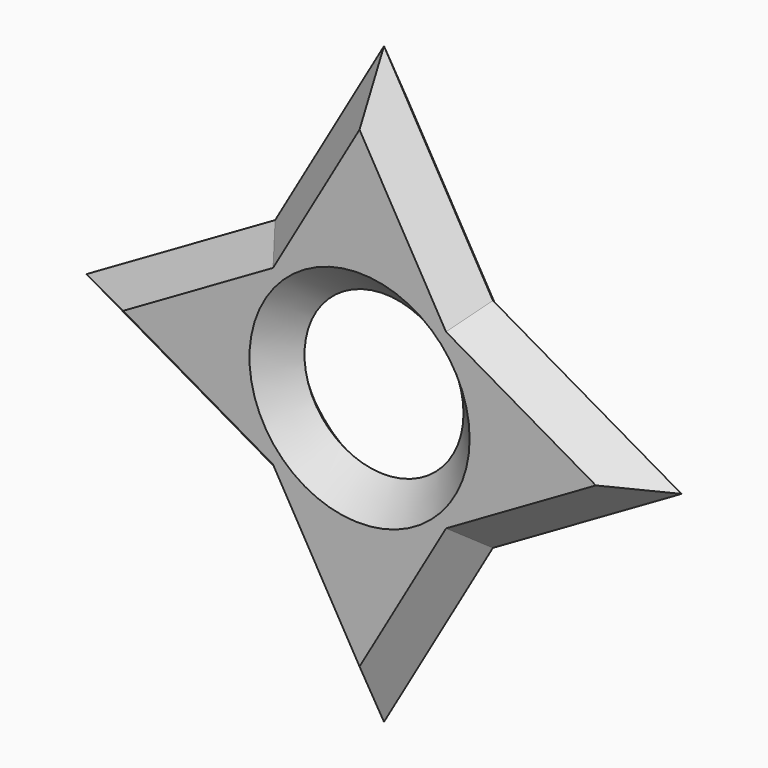
from build123d import *

# Parameters (mm, degrees)
F0_W         = 25.4
F0_H         = 25.4
F0_R         = 6.35
F1_DEPTH     = 6.35
F2_SIZE      = 5.08
F3_T4_DEPTH  = 51.5282991577
F3_T9_DEPTH  = 51.5282991577
F3_T14_DEPTH = 51.5282991577
F3_T19_DEPTH = 51.5282991577
F3_T24_DEPTH = 51.5282991577
F3_T29_DEPTH = 51.5282991577
F3_T34_DEPTH = 51.5282991577
F3_T39_DEPTH = 51.5282991577
F3_T47_DEPTH = 51.5282991577
F3_T51_DEPTH = 51.5282991577
F3_T58_DEPTH = 51.5282991577
F3_T62_DEPTH = 51.5282991577
F3_T69_DEPTH = 51.5282991577
F3_T73_DEPTH = 51.5282991577
F3_T80_DEPTH = 51.5282991577
F3_T84_DEPTH = 51.5282991577


# Not quite as in the source:
# - a fillet or chamfer that OpenCascade refuses, or shapes differently, is made with other operations: its cross-section is extruded or revolved along the edge and cut away or added


with BuildPart() as f1:
    # F0 (on Front) → F1 (new body)
    with BuildSketch(Plane.XZ):
        with Locations((12.7, 12.7)):
            Rectangle(F0_W, F0_H)
        with Locations((12.7, 12.7)):
            Circle(F0_R, mode=Mode.SUBTRACT)
        Polygon((12.7, 47.3970452561), (0, 25.4), (25.4, 25.4), align=None)
        Polygon((-21.9970452561, 12.7), (0, 0), (0, 25.4), align=None)
        Polygon((25.4, 25.4), (25.4, 0), (47.3970452561, 12.7), align=None)
        Polygon((25.4, 0), (0, 0), (12.7, -21.9970452561), align=None)
    extrude(amount=F1_DEPTH)

    # F2
    f2_edges = [f1.edges().sort_by_distance(p)[0] for p in [
        (36.398523, -6.35, 6.35),
        (36.398523, -6.35, 19.05),
        (19.05, -6.35, 36.398523),
        (6.35, -6.35, 36.398523),
        (-10.998523, -6.35, 19.05),
        (-10.998523, -6.35, 6.35),
        (6.35, -6.35, -10.998523),
        (19.05, -6.35, -10.998523),
        (6.35, -6.35, 12.7),
    ]]
    chamfer(f2_edges, length=F2_SIZE)

    # F3: chamfer of 5.08 on 9 edges, made by hand


with BuildPart() as f3_tool2:
    # F3_s3 → F3_t4 (new body)
    with BuildSketch(Plane(origin=(7.7361145859, 0, 4.4664478386), x_dir=(0, 1, 0), z_dir=(0.8660254038, 0, 0.5))):
        Polygon((-5.08, -12.7), (0, -7.62), (0, -12.7), align=None)
    extrude(amount=F3_T4_DEPTH)

    split(bisect_by=Plane(origin=(19.05, 0, -10.9985226281), x_dir=(0, 1, 0), z_dir=(0.8660254038, 0, -0.5)), keep=Keep.TOP)


with BuildPart() as f1_1:
    add(f1.part)

    # F3_t1: cut F3_tool2
    add(f3_tool2.part, mode=Mode.SUBTRACT)


with BuildPart() as f3_tool7:
    # F3_s8 → F3_t9 (new body)
    with BuildSketch(Plane(origin=(41.3624080422, 0, -23.8805974175), x_dir=(0, 1, 0), z_dir=(-0.8660254038, 0, 0.5))):
        Polygon((0, -29.6170452561), (-5.08, -34.6970452561), (0, -34.6970452561), align=None)
    extrude(amount=F3_T9_DEPTH)

    split(bisect_by=Plane(origin=(30.0485226281, 0, 17.3485226281), x_dir=(0, 1, 0), z_dir=(0.8660254038, 0, 0.5)), keep=Keep.TOP)


with BuildPart() as f1_2:
    add(f1_1.part)

    # F3_t6: cut F3_tool7
    add(f3_tool7.part, mode=Mode.SUBTRACT)


with BuildPart() as f3_tool12:
    # F3_s13 → F3_t14 (new body)
    with BuildSketch(Plane(origin=(1.8835521614, 0, -3.2624080422), x_dir=(0, 1, 0), z_dir=(-0.5, 0, 0.8660254038))):
        Polygon((0, -29.6170452561), (-5.08, -34.6970452561), (0, -34.6970452561), align=None)
    extrude(amount=F3_T14_DEPTH)

    split(bisect_by=Plane(origin=(17.3485226281, 0, 30.0485226281), x_dir=(0, 1, 0), z_dir=(0.5, 0, 0.8660254038)), keep=Keep.TOP)


with BuildPart() as f1_3:
    add(f1_2.part)

    # F3_t11: cut F3_tool12
    add(f3_tool12.part, mode=Mode.SUBTRACT)


with BuildPart() as f3_tool17:
    # F3_s18 → F3_t19 (new body)
    with BuildSketch(Plane(origin=(30.2305974175, 0, 52.3609306703), x_dir=(0, 1, 0), z_dir=(-0.5, 0, -0.8660254038))):
        Polygon((0, -7.62), (-5.08, -12.7), (0, -12.7), align=None)
    extrude(amount=F3_T19_DEPTH)

    split(bisect_by=Plane(origin=(-10.9985226281, 0, 19.05), x_dir=(0, 1, 0), z_dir=(-0.5, 0, 0.8660254038)), keep=Keep.TOP)


with BuildPart() as f1_4:
    add(f1_3.part)

    # F3_t16: cut F3_tool17
    add(f3_tool17.part, mode=Mode.SUBTRACT)


with BuildPart() as f3_tool22:
    # F3_s23 → F3_t24 (new body)
    with BuildSketch(Plane(origin=(22.3124080422, 0, 12.8820747894), x_dir=(0, 1, 0), z_dir=(-0.8660254038, 0, -0.5))):
        Polygon((0, -16.9170452561), (-5.08, -21.9970452561), (0, -21.9970452561), align=None)
    extrude(amount=F3_T24_DEPTH)

    split(bisect_by=Plane(origin=(-10.9985226281, 0, 6.35), x_dir=(0, 1, 0), z_dir=(-0.8660254038, 0, 0.5)), keep=Keep.TOP)


with BuildPart() as f1_5:
    add(f1_4.part)

    # F3_t21: cut F3_tool22
    add(f3_tool22.part, mode=Mode.SUBTRACT)


with BuildPart() as f3_tool27:
    # F3_s28 → F3_t29 (new body)
    with BuildSketch(Plane(origin=(-33.3109306703, 0, 19.2320747894), x_dir=(0, 1, 0), z_dir=(0.8660254038, 0, -0.5))):
        Polygon((0, 5.08), (-5.08, 0), (0, 0), align=None)
    extrude(amount=F3_T29_DEPTH)

    split(bisect_by=Plane(origin=(0, 0, 0), x_dir=(0, 1, 0), z_dir=(-0.8660254038, 0, -0.5)), keep=Keep.TOP)


with BuildPart() as f1_6:
    add(f1_5.part)

    # F3_t26: cut F3_tool27
    add(f3_tool27.part, mode=Mode.SUBTRACT)


with BuildPart() as f3_tool32:
    # F3_s33 → F3_t34 (new body)
    with BuildSketch(Plane(origin=(-6.5320747894, 0, 11.3138854141), x_dir=(0, 1, 0), z_dir=(0.5, 0, -0.8660254038))):
        Polygon((0, 5.08), (-5.08, 0), (0, 0), align=None)
    extrude(amount=F3_T34_DEPTH)

    split(bisect_by=Plane(origin=(0, 0, 0), x_dir=(0, 1, 0), z_dir=(-0.5, 0, -0.8660254038)), keep=Keep.TOP)


with BuildPart() as f1_7:
    add(f1_6.part)

    # F3_t31: cut F3_tool32
    add(f3_tool32.part, mode=Mode.SUBTRACT)


with BuildPart() as f3_tool37:
    # F3_s38 → F3_t39 (new body)
    with BuildSketch(Plane(origin=(-12.8820747894, 0, -22.3124080422), x_dir=(0, 1, 0), z_dir=(0.5, 0, 0.8660254038))):
        Polygon((-5.08, -21.9970452561), (0, -16.9170452561), (0, -21.9970452561), align=None)
    extrude(amount=F3_T39_DEPTH)

    split(bisect_by=Plane(origin=(6.35, 0, -10.9985226281), x_dir=(0, 1, 0), z_dir=(0.5, 0, -0.8660254038)), keep=Keep.TOP)


with BuildPart() as f1_8:
    add(f1_7.part)

    # F3_t36: cut F3_tool37
    add(f3_tool37.part, mode=Mode.SUBTRACT)

    # F3_s41 → F3_t42 (revolve, cut)
    with BuildSketch(Plane.XY.offset(12.7)):
        Polygon((24.13, 0), (19.05, -5.08), (19.05, 0), align=None)
    revolve(axis=Axis((12.7, 0, 12.7), (0, -1, 0)), mode=Mode.SUBTRACT)


with BuildPart() as f3_tool45:
    # F3_s46 → F3_t47 (new body)
    with BuildSketch(Plane(origin=(7.7361145859, 0, 4.4664478386), x_dir=(0, 1, 0), z_dir=(0.8660254038, 0, 0.5))):
        Polygon((-5.08, -12.7), (0, -7.62), (0, -12.7), align=None)
    extrude(amount=F3_T47_DEPTH)

    split(bisect_by=Plane(origin=(19.05, 0, -10.9985226281), x_dir=(0, 1, 0), z_dir=(-0.8660254038, 0, 0.5)), keep=Keep.TOP)


with BuildPart() as f3_tool49:
    # F3_s50 → F3_t51 (new body)
    with BuildSketch(Plane(origin=(-12.8820747894, 0, -22.3124080422), x_dir=(0, 1, 0), z_dir=(0.5, 0, 0.8660254038))):
        Polygon((-5.08, -21.9970452561), (0, -16.9170452561), (0, -21.9970452561), align=None)
    extrude(amount=F3_T51_DEPTH)

    split(bisect_by=Plane(origin=(6.35, 0, -10.9985226281), x_dir=(0, 1, 0), z_dir=(-0.5, 0, 0.8660254038)), keep=Keep.TOP)


with BuildPart() as f3_tool45_1:
    add(f3_tool45.part)

    # F3_t53: intersect F3_tool49
    add(f3_tool49.part, mode=Mode.INTERSECT)


with BuildPart() as f1_9:
    add(f1_8.part)

    # F3_t43: cut F3_tool45
    add(f3_tool45_1.part, mode=Mode.SUBTRACT)


with BuildPart() as f3_tool56:
    # F3_s57 → F3_t58 (new body)
    with BuildSketch(Plane(origin=(41.3624080422, 0, -23.8805974175), x_dir=(0, 1, 0), z_dir=(-0.8660254038, 0, 0.5))):
        Polygon((0, -29.6170452561), (-5.08, -34.6970452561), (0, -34.6970452561), align=None)
    extrude(amount=F3_T58_DEPTH)

    split(bisect_by=Plane(origin=(30.0485226281, 0, 17.3485226281), x_dir=(0, 1, 0), z_dir=(-0.8660254038, 0, -0.5)), keep=Keep.TOP)


with BuildPart() as f3_tool60:
    # F3_s61 → F3_t62 (new body)
    with BuildSketch(Plane(origin=(1.8835521614, 0, -3.2624080422), x_dir=(0, 1, 0), z_dir=(-0.5, 0, 0.8660254038))):
        Polygon((0, -29.6170452561), (-5.08, -34.6970452561), (0, -34.6970452561), align=None)
    extrude(amount=F3_T62_DEPTH)

    split(bisect_by=Plane(origin=(17.3485226281, 0, 30.0485226281), x_dir=(0, 1, 0), z_dir=(-0.5, 0, -0.8660254038)), keep=Keep.TOP)


with BuildPart() as f3_tool56_1:
    add(f3_tool56.part)

    # F3_t64: intersect F3_tool60
    add(f3_tool60.part, mode=Mode.INTERSECT)


with BuildPart() as f1_10:
    add(f1_9.part)

    # F3_t54: cut F3_tool56
    add(f3_tool56_1.part, mode=Mode.SUBTRACT)


with BuildPart() as f3_tool67:
    # F3_s68 → F3_t69 (new body)
    with BuildSketch(Plane(origin=(30.2305974175, 0, 52.3609306703), x_dir=(0, 1, 0), z_dir=(-0.5, 0, -0.8660254038))):
        Polygon((0, -7.62), (-5.08, -12.7), (0, -12.7), align=None)
    extrude(amount=F3_T69_DEPTH)

    split(bisect_by=Plane(origin=(-10.9985226281, 0, 19.05), x_dir=(0, 1, 0), z_dir=(0.5, 0, -0.8660254038)), keep=Keep.TOP)


with BuildPart() as f3_tool71:
    # F3_s72 → F3_t73 (new body)
    with BuildSketch(Plane(origin=(22.3124080422, 0, 12.8820747894), x_dir=(0, 1, 0), z_dir=(-0.8660254038, 0, -0.5))):
        Polygon((0, -16.9170452561), (-5.08, -21.9970452561), (0, -21.9970452561), align=None)
    extrude(amount=F3_T73_DEPTH)

    split(bisect_by=Plane(origin=(-10.9985226281, 0, 6.35), x_dir=(0, 1, 0), z_dir=(0.8660254038, 0, -0.5)), keep=Keep.TOP)


with BuildPart() as f3_tool67_1:
    add(f3_tool67.part)

    # F3_t75: intersect F3_tool71
    add(f3_tool71.part, mode=Mode.INTERSECT)


with BuildPart() as f1_11:
    add(f1_10.part)

    # F3_t65: cut F3_tool67
    add(f3_tool67_1.part, mode=Mode.SUBTRACT)


with BuildPart() as f3_tool78:
    # F3_s79 → F3_t80 (new body)
    with BuildSketch(Plane(origin=(-33.3109306703, 0, 19.2320747894), x_dir=(0, 1, 0), z_dir=(0.8660254038, 0, -0.5))):
        Polygon((0, 5.08), (-5.08, 0), (0, 0), align=None)
    extrude(amount=F3_T80_DEPTH)

    split(bisect_by=Plane(origin=(0, 0, 0), x_dir=(0, 1, 0), z_dir=(0.8660254038, 0, 0.5)), keep=Keep.TOP)


with BuildPart() as f3_tool82:
    # F3_s83 → F3_t84 (new body)
    with BuildSketch(Plane(origin=(-6.5320747894, 0, 11.3138854141), x_dir=(0, 1, 0), z_dir=(0.5, 0, -0.8660254038))):
        Polygon((0, 5.08), (-5.08, 0), (0, 0), align=None)
    extrude(amount=F3_T84_DEPTH)

    split(bisect_by=Plane(origin=(0, 0, 0), x_dir=(0, 1, 0), z_dir=(0.5, 0, 0.8660254038)), keep=Keep.TOP)


with BuildPart() as f3_tool78_1:
    add(f3_tool78.part)

    # F3_t86: intersect F3_tool82
    add(f3_tool82.part, mode=Mode.INTERSECT)


with BuildPart() as f1_12:
    add(f1_11.part)

    # F3_t76: cut F3_tool78
    add(f3_tool78_1.part, mode=Mode.SUBTRACT)


solid = f1_12.part
